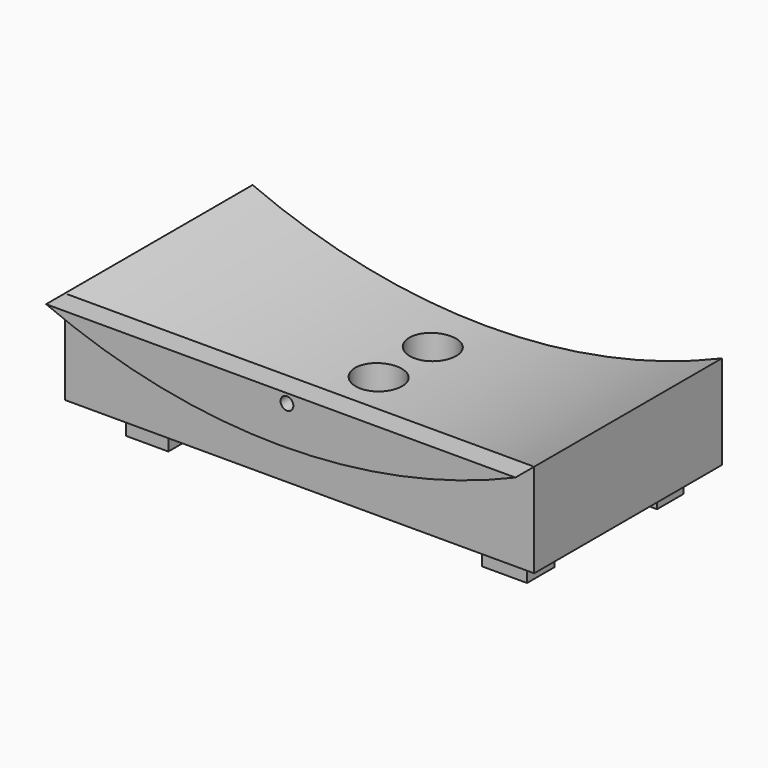
from build123d import *

# Parameters (mm, degrees)
F1_DEPTH  = 50
F2_R      = 5
F3_DEPTH  = 25
F3_FACE_R = 5
F4_DEPTH  = 143
F5_DEPTH  = 25.0010001
F6_W      = 7.0818345994
F6_H      = 5.9487447143
F7_DEPTH  = 6
F6_W_2    = 9.9145658314
F6_H_2    = 7.0818341337
F6_W_3    = 8.7814740837
F11_DEPTH = 5
F12_R     = 1.2416871231
F13_DEPTH = 146
F14_R     = 1.3622183524
F15_DEPTH = 33.4
F16_W     = 9.0647470206
F16_H     = 7.6483786106
F16_W_2   = 9.6312910318
F16_H_2   = 7.3651075363
F17_DEPTH = 6


# Not quite as in the source:
# - an extrude ends at something that could not be found from the text; its depth is read off the source's solid


with BuildPart() as f1:
    # F0 (on Front) → F1 (new body)
    with BuildSketch(Plane.XZ):
        with BuildLine():
            Line((-40.7999969139, 20), (-40.7999969139, 0))
            Line((-40.7999969139, 0), (59.2000030861, 0))
            Line((59.2000030861, 0), (59.2000030861, 20))
            ThreePointArc((59.2000030861, 20), (9.2000030861, 9.7404933021), (-40.7999969139, 20))
        make_face()
    extrude(amount=F1_DEPTH)

    # F2 (on Top) → F3 (join)
    with BuildSketch(Plane.XY):
        with Locations((6.8606630445, -11.5833937097)):
            Circle(F2_R)
        with Locations((6.6326826697, -25.7181784424)):
            Circle(F2_R)
        with Locations((5.9487419203, -40.5368994273)):
            Circle(F2_R)
    extrude(amount=F3_DEPTH)

    # F2 (on Top) + F3_face (on face) → F4 (cut, through all)
    with BuildSketch(Plane.XY):
        with Locations((6.8606630445, -11.5833937097)):
            Circle(F2_R)
        with Locations((6.6326826697, -25.7181784424)):
            Circle(F2_R)
        with Locations((5.9487419203, -40.5368994273)):
            Circle(F2_R)
    with BuildSketch(Plane(origin=(6.6326826697, -25.7181784424, 25), x_dir=(1, 0, 0), z_dir=(0, 0, 1))):
        Circle(F3_FACE_R)
        with Locations((-0.6839407494, -14.8187209849)):
            Circle(F3_FACE_R)
    extrude(amount=-F4_DEPTH, mode=Mode.SUBTRACT)

    # F5 (cut, through all): a face of the model
    f5_faces = [f1.faces().sort_by_distance(p)[0] for p in [
        (6.8606630445, -11.5833937097, 25),
    ]]
    extrude(f5_faces, amount=-F5_DEPTH, mode=Mode.SUBTRACT)

    # F6 (on Top) → F7, piece 3 (join)
    with BuildSketch(Plane.XY):
        with Locations((48.581385985, -6.6569244955)):
            Rectangle(F6_W_2, F6_H_2)
        with Locations((-27.6191551238, -6.6569244955)):
            Rectangle(F6_W_3, F6_H_2)
    extrude(amount=-F7_DEPTH)

    # F12 (on Front) → F13 (cut, through all)
    with BuildSketch(Plane.XZ):
        with Locations((3.8911467418, 17.7770014852)):
            Circle(F12_R)
    extrude(amount=-F13_DEPTH, mode=Mode.SUBTRACT)

    # F16 (on face) → F17 (join)
    with BuildSketch(Plane(origin=(0, 0, 0), x_dir=(1, 0, 0), z_dir=(0, 0, -1))):
        with Locations((-27.4775186554, 40.9330055118)):
            Rectangle(F16_W, F16_H)
        with Locations((48.4397485852, 40.7913699746)):
            Rectangle(F16_W_2, F16_H_2)
    extrude(amount=F17_DEPTH)


with BuildPart() as f7:
    # F6 (on Top) → F7 (new body)
    with BuildSketch(Plane.XY):
        with Locations((-26.7693353817, -55.3799495101)):
            Rectangle(F6_W, F6_H)
    extrude(amount=-F7_DEPTH)


with BuildPart() as f7b:
    # F6 (on Top) → F7, piece 2 (new body)
    with BuildSketch(Plane.XY):
        with Locations((48.581385985, -55.3799495101)):
            Rectangle(F6_W_2, F6_H)
    extrude(amount=-F7_DEPTH)


with BuildPart() as f11:
    # F10 (on face) → F11 (new body)
    with BuildSketch(Plane.XZ.offset(50)):
        with BuildLine():
            Line((59.2000030861, 20), (-40.7999969139, 20))
            ThreePointArc((-40.7999969139, 20), (9.2000030861, 9.7404933021), (59.2000030861, 20))
        make_face()
    extrude(amount=F11_DEPTH)

    # F14 (on face) → F15 (cut)
    with BuildSketch(Plane(origin=(0, -50, 0), x_dir=(-1, 0, 0), z_dir=(0, 1, 0))):
        with Locations((-10.5227353051, 18.0770270526)):
            Circle(F14_R)
    extrude(amount=-F15_DEPTH, mode=Mode.SUBTRACT)


solid = Compound([f1.part, f11.part])
